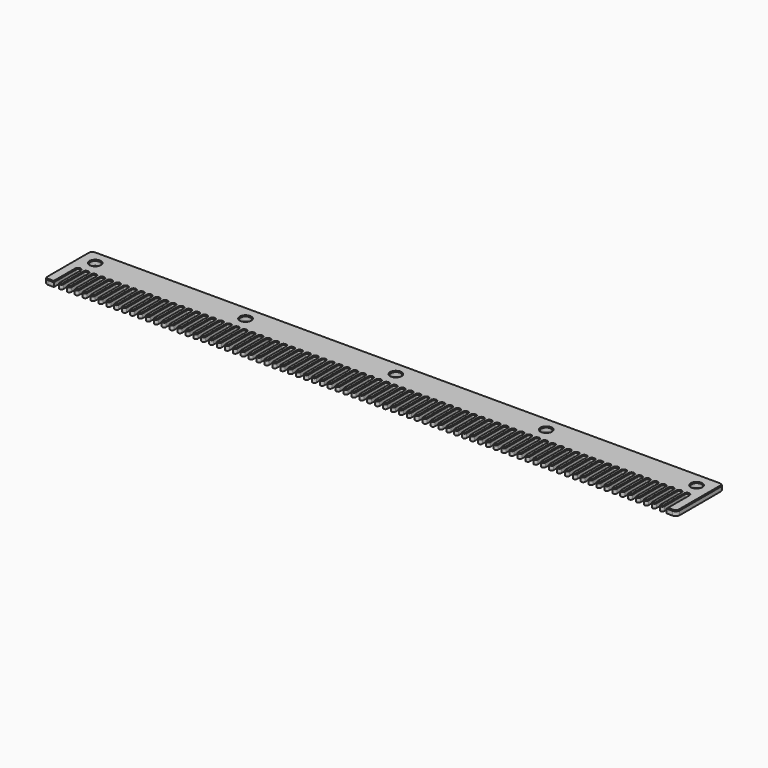
from build123d import *

# Parameters (mm, degrees)
F0_R     = 1.5875
F1_DEPTH = 1.5875
F2_SIZE  = 0.254


# Not quite as in the source:
# - a length typed as a fraction of an inch, garbled in the dataset ("3 / 203.2 mm" for 3/8 in), is restored


with BuildPart() as f1:
    # F0 (on Top) → F1 (new body)
    with BuildSketch(Plane.XY):
        with BuildLine():
            ThreePointArc((101.6, 8.2549999998), (101.2280256121, 9.1530256119), (100.33, 9.5249999998))
            Line((100.33, 9.5249999998), (-100.33, 9.5250000002))
            ThreePointArc((-100.33, 9.5250000002), (-101.2280256121, 9.1530256123), (-101.6, 8.2550000002))
            Line((-101.6, 8.2550000002), (-101.6, -8.255))
            ThreePointArc((-101.6, -8.255), (-101.2280256121, -9.1530256121), (-100.33, -9.525))
            Line((-100.33, -9.525), (-98.425, -9.525))
            Line((-98.425, -9.525), (-98.425, -0.635))
            ThreePointArc((-98.425, -0.635), (-97.79, 0), (-97.155, -0.635))
            Line((-97.155, -0.635), (-97.155, -8.89))
            ThreePointArc((-97.155, -8.89), (-96.52, -9.525), (-95.885, -8.89))
            Line((-95.885, -8.89), (-95.885, -0.635))
            ThreePointArc((-95.885, -0.635), (-95.25, 0), (-94.615, -0.635))
            Line((-94.615, -0.635), (-94.615, -8.89))
            ThreePointArc((-94.615, -8.89), (-93.98, -9.525), (-93.345, -8.89))
            Line((-93.345, -8.89), (-93.345, -0.635))
            ThreePointArc((-93.345, -0.635), (-92.71, 0), (-92.075, -0.635))
            Line((-92.075, -0.635), (-92.075, -8.89))
            ThreePointArc((-92.075, -8.89), (-91.44, -9.525), (-90.805, -8.89))
            Line((-90.805, -8.89), (-90.805, -0.635))
            ThreePointArc((-90.805, -0.635), (-90.17, 0), (-89.535, -0.635))
            Line((-89.535, -0.635), (-89.535, -8.89))
            ThreePointArc((-89.535, -8.89), (-88.9, -9.525), (-88.265, -8.89))
            Line((-88.265, -8.89), (-88.265, -0.635))
            ThreePointArc((-88.265, -0.635), (-87.63, 0), (-86.995, -0.635))
            Line((-86.995, -0.635), (-86.995, -8.89))
            ThreePointArc((-86.995, -8.89), (-86.36, -9.525), (-85.725, -8.89))
            Line((-85.725, -8.89), (-85.725, -0.635))
            ThreePointArc((-85.725, -0.635), (-85.09, 0), (-84.455, -0.635))
            Line((-84.455, -0.635), (-84.455, -8.89))
            ThreePointArc((-84.455, -8.89), (-83.82, -9.525), (-83.185, -8.89))
            Line((-83.185, -8.89), (-83.185, -0.635))
            ThreePointArc((-83.185, -0.635), (-82.55, 0), (-81.915, -0.635))
            Line((-81.915, -0.635), (-81.915, -8.89))
            ThreePointArc((-81.915, -8.89), (-81.28, -9.525), (-80.645, -8.89))
            Line((-80.645, -8.89), (-80.645, -0.635))
            ThreePointArc((-80.645, -0.635), (-80.01, 0), (-79.375, -0.635))
            Line((-79.375, -0.635), (-79.375, -8.89))
            ThreePointArc((-79.375, -8.89), (-78.74, -9.525), (-78.105, -8.89))
            Line((-78.105, -8.89), (-78.105, -0.635))
            ThreePointArc((-78.105, -0.635), (-77.47, 0), (-76.835, -0.635))
            Line((-76.835, -0.635), (-76.835, -8.89))
            ThreePointArc((-76.835, -8.89), (-76.2, -9.525), (-75.565, -8.89))
            Line((-75.565, -8.89), (-75.565, -0.635))
            ThreePointArc((-75.565, -0.635), (-74.93, 0), (-74.295, -0.635))
            Line((-74.295, -0.635), (-74.295, -8.89))
            ThreePointArc((-74.295, -8.89), (-73.66, -9.525), (-73.025, -8.89))
            Line((-73.025, -8.89), (-73.025, -0.635))
            ThreePointArc((-73.025, -0.635), (-72.39, 0), (-71.755, -0.635))
            Line((-71.755, -0.635), (-71.755, -8.89))
            ThreePointArc((-71.755, -8.89), (-71.12, -9.525), (-70.485, -8.89))
            Line((-70.485, -8.89), (-70.485, -0.635))
            ThreePointArc((-70.485, -0.635), (-69.85, 0), (-69.215, -0.635))
            Line((-69.215, -0.635), (-69.215, -8.89))
            ThreePointArc((-69.215, -8.89), (-68.58, -9.525), (-67.945, -8.89))
            Line((-67.945, -8.89), (-67.945, -0.635))
            ThreePointArc((-67.945, -0.635), (-67.31, 0), (-66.675, -0.635))
            Line((-66.675, -0.635), (-66.675, -8.89))
            ThreePointArc((-66.675, -8.89), (-66.04, -9.525), (-65.405, -8.89))
            Line((-65.405, -8.89), (-65.405, -0.635))
            ThreePointArc((-65.405, -0.635), (-64.77, 0), (-64.135, -0.635))
            Line((-64.135, -0.635), (-64.135, -8.89))
            ThreePointArc((-64.135, -8.89), (-63.5, -9.525), (-62.865, -8.89))
            Line((-62.865, -8.89), (-62.865, -0.635))
            ThreePointArc((-62.865, -0.635), (-62.23, 0), (-61.595, -0.635))
            Line((-61.595, -0.635), (-61.595, -8.89))
            ThreePointArc((-61.595, -8.89), (-60.96, -9.525), (-60.325, -8.89))
            Line((-60.325, -8.89), (-60.325, -0.635))
            ThreePointArc((-60.325, -0.635), (-59.69, 0), (-59.055, -0.635))
            Line((-59.055, -0.635), (-59.055, -8.89))
            ThreePointArc((-59.055, -8.89), (-58.42, -9.525), (-57.785, -8.89))
            Line((-57.785, -8.89), (-57.785, -0.635))
            ThreePointArc((-57.785, -0.635), (-57.15, 0), (-56.515, -0.635))
            Line((-56.515, -0.635), (-56.515, -8.89))
            ThreePointArc((-56.515, -8.89), (-55.88, -9.525), (-55.245, -8.89))
            Line((-55.245, -8.89), (-55.245, -0.635))
            ThreePointArc((-55.245, -0.635), (-54.61, 0), (-53.975, -0.635))
            Line((-53.975, -0.635), (-53.975, -8.89))
            ThreePointArc((-53.975, -8.89), (-53.34, -9.525), (-52.705, -8.89))
            Line((-52.705, -8.89), (-52.705, -0.635))
            ThreePointArc((-52.705, -0.635), (-52.07, 0), (-51.435, -0.635))
            Line((-51.435, -0.635), (-51.435, -8.89))
            ThreePointArc((-51.435, -8.89), (-50.8, -9.525), (-50.165, -8.89))
            Line((-50.165, -8.89), (-50.165, -0.635))
            ThreePointArc((-50.165, -0.635), (-49.53, 0), (-48.895, -0.635))
            Line((-48.895, -0.635), (-48.895, -8.89))
            ThreePointArc((-48.895, -8.89), (-48.26, -9.525), (-47.625, -8.89))
            Line((-47.625, -8.89), (-47.625, -0.635))
            ThreePointArc((-47.625, -0.635), (-46.99, 0), (-46.355, -0.635))
            Line((-46.355, -0.635), (-46.355, -8.89))
            ThreePointArc((-46.355, -8.89), (-45.72, -9.525), (-45.085, -8.89))
            Line((-45.085, -8.89), (-45.085, -0.635))
            ThreePointArc((-45.085, -0.635), (-44.45, 0), (-43.815, -0.635))
            Line((-43.815, -0.635), (-43.815, -8.89))
            ThreePointArc((-43.815, -8.89), (-43.18, -9.525), (-42.545, -8.89))
            Line((-42.545, -8.89), (-42.545, -0.635))
            ThreePointArc((-42.545, -0.635), (-41.91, 0), (-41.275, -0.635))
            Line((-41.275, -0.635), (-41.275, -8.89))
            ThreePointArc((-41.275, -8.89), (-40.64, -9.525), (-40.005, -8.89))
            Line((-40.005, -8.89), (-40.005, -0.635))
            ThreePointArc((-40.005, -0.635), (-39.37, 0), (-38.735, -0.635))
            Line((-38.735, -0.635), (-38.735, -8.89))
            ThreePointArc((-38.735, -8.89), (-38.1, -9.525), (-37.465, -8.89))
            Line((-37.465, -8.89), (-37.465, -0.635))
            ThreePointArc((-37.465, -0.635), (-36.83, 0), (-36.195, -0.635))
            Line((-36.195, -0.635), (-36.195, -8.89))
            ThreePointArc((-36.195, -8.89), (-35.56, -9.525), (-34.925, -8.89))
            Line((-34.925, -8.89), (-34.925, -0.635))
            ThreePointArc((-34.925, -0.635), (-34.29, 0), (-33.655, -0.635))
            Line((-33.655, -0.635), (-33.655, -8.89))
            ThreePointArc((-33.655, -8.89), (-33.02, -9.525), (-32.385, -8.89))
            Line((-32.385, -8.89), (-32.385, -0.635))
            ThreePointArc((-32.385, -0.635), (-31.75, 0), (-31.115, -0.635))
            Line((-31.115, -0.635), (-31.115, -8.89))
            ThreePointArc((-31.115, -8.89), (-30.48, -9.525), (-29.845, -8.89))
            Line((-29.845, -8.89), (-29.845, -0.635))
            ThreePointArc((-29.845, -0.635), (-29.21, 0), (-28.575, -0.635))
            Line((-28.575, -0.635), (-28.575, -8.89))
            ThreePointArc((-28.575, -8.89), (-27.94, -9.525), (-27.305, -8.89))
            Line((-27.305, -8.89), (-27.305, -0.635))
            ThreePointArc((-27.305, -0.635), (-26.67, 0), (-26.035, -0.635))
            Line((-26.035, -0.635), (-26.035, -8.89))
            ThreePointArc((-26.035, -8.89), (-25.4, -9.525), (-24.765, -8.89))
            Line((-24.765, -8.89), (-24.765, -0.635))
            ThreePointArc((-24.765, -0.635), (-24.13, 0), (-23.495, -0.635))
            Line((-23.495, -0.635), (-23.495, -8.89))
            ThreePointArc((-23.495, -8.89), (-22.86, -9.525), (-22.225, -8.89))
            Line((-22.225, -8.89), (-22.225, -0.635))
            ThreePointArc((-22.225, -0.635), (-21.59, 0), (-20.955, -0.635))
            Line((-20.955, -0.635), (-20.955, -8.89))
            ThreePointArc((-20.955, -8.89), (-20.32, -9.525), (-19.685, -8.89))
            Line((-19.685, -8.89), (-19.685, -0.635))
            ThreePointArc((-19.685, -0.635), (-19.05, 0), (-18.415, -0.635))
            Line((-18.415, -0.635), (-18.415, -8.89))
            ThreePointArc((-18.415, -8.89), (-17.78, -9.525), (-17.145, -8.89))
            Line((-17.145, -8.89), (-17.145, -0.635))
            ThreePointArc((-17.145, -0.635), (-16.51, 0), (-15.875, -0.635))
            Line((-15.875, -0.635), (-15.875, -8.89))
            ThreePointArc((-15.875, -8.89), (-15.24, -9.525), (-14.605, -8.89))
            Line((-14.605, -8.89), (-14.605, -0.635))
            ThreePointArc((-14.605, -0.635), (-13.97, 0), (-13.335, -0.635))
            Line((-13.335, -0.635), (-13.335, -8.89))
            ThreePointArc((-13.335, -8.89), (-12.7, -9.525), (-12.065, -8.89))
            Line((-12.065, -8.89), (-12.065, -0.635))
            ThreePointArc((-12.065, -0.635), (-11.43, 0), (-10.795, -0.635))
            Line((-10.795, -0.635), (-10.795, -8.89))
            ThreePointArc((-10.795, -8.89), (-10.16, -9.525), (-9.525, -8.89))
            Line((-9.525, -8.89), (-9.525, -0.635))
            ThreePointArc((-9.525, -0.635), (-8.89, 0), (-8.255, -0.635))
            Line((-8.255, -0.635), (-8.255, -8.89))
            ThreePointArc((-8.255, -8.89), (-7.62, -9.525), (-6.985, -8.89))
            Line((-6.985, -8.89), (-6.985, -0.635))
            ThreePointArc((-6.985, -0.635), (-6.35, 0), (-5.715, -0.635))
            Line((-5.715, -0.635), (-5.715, -8.89))
            ThreePointArc((-5.715, -8.89), (-5.08, -9.525), (-4.445, -8.89))
            Line((-4.445, -8.89), (-4.445, -0.635))
            ThreePointArc((-4.445, -0.635), (-3.81, 0), (-3.175, -0.635))
            Line((-3.175, -0.635), (-3.175, -8.89))
            ThreePointArc((-3.175, -8.89), (-2.54, -9.525), (-1.905, -8.89))
            Line((-1.905, -8.89), (-1.905, -0.635))
            ThreePointArc((-1.905, -0.635), (-1.27, 0), (-0.635, -0.635))
            Line((-0.635, -0.635), (-0.635, -8.89))
            ThreePointArc((-0.635, -8.89), (0, -9.525), (0.635, -8.89))
            Line((0.635, -8.89), (0.635, -0.635))
            ThreePointArc((0.635, -0.635), (1.27, 0), (1.905, -0.635))
            Line((1.905, -0.635), (1.905, -8.89))
            ThreePointArc((1.905, -8.89), (2.54, -9.525), (3.175, -8.89))
            Line((3.175, -8.89), (3.175, -0.635))
            ThreePointArc((3.175, -0.635), (3.81, 0), (4.445, -0.635))
            Line((4.445, -0.635), (4.445, -8.89))
            ThreePointArc((4.445, -8.89), (5.08, -9.525), (5.715, -8.89))
            Line((5.715, -8.89), (5.715, -0.635))
            ThreePointArc((5.715, -0.635), (6.35, 0), (6.985, -0.635))
            Line((6.985, -0.635), (6.985, -8.89))
            ThreePointArc((6.985, -8.89), (7.62, -9.525), (8.255, -8.89))
            Line((8.255, -8.89), (8.255, -0.635))
            ThreePointArc((8.255, -0.635), (8.89, 0), (9.525, -0.635))
            Line((9.525, -0.635), (9.525, -8.89))
            ThreePointArc((9.525, -8.89), (10.16, -9.525), (10.795, -8.89))
            Line((10.795, -8.89), (10.795, -0.635))
            ThreePointArc((10.795, -0.635), (11.43, 0), (12.065, -0.635))
            Line((12.065, -0.635), (12.065, -8.89))
            ThreePointArc((12.065, -8.89), (12.7, -9.525), (13.335, -8.89))
            Line((13.335, -8.89), (13.335, -0.635))
            ThreePointArc((13.335, -0.635), (13.97, 0), (14.605, -0.635))
            Line((14.605, -0.635), (14.605, -8.89))
            ThreePointArc((14.605, -8.89), (15.24, -9.525), (15.875, -8.89))
            Line((15.875, -8.89), (15.875, -0.635))
            ThreePointArc((15.875, -0.635), (16.51, 0), (17.145, -0.635))
            Line((17.145, -0.635), (17.145, -8.89))
            ThreePointArc((17.145, -8.89), (17.78, -9.525), (18.415, -8.89))
            Line((18.415, -8.89), (18.415, -0.635))
            ThreePointArc((18.415, -0.635), (19.05, 0), (19.685, -0.635))
            Line((19.685, -0.635), (19.685, -8.89))
            ThreePointArc((19.685, -8.89), (20.32, -9.525), (20.955, -8.89))
            Line((20.955, -8.89), (20.955, -0.635))
            ThreePointArc((20.955, -0.635), (21.59, 0), (22.225, -0.635))
            Line((22.225, -0.635), (22.225, -8.89))
            ThreePointArc((22.225, -8.89), (22.86, -9.525), (23.495, -8.89))
            Line((23.495, -8.89), (23.495, -0.635))
            ThreePointArc((23.495, -0.635), (24.13, 0), (24.765, -0.635))
            Line((24.765, -0.635), (24.765, -8.89))
            ThreePointArc((24.765, -8.89), (25.4, -9.525), (26.035, -8.89))
            Line((26.035, -8.89), (26.035, -0.635))
            ThreePointArc((26.035, -0.635), (26.67, 0), (27.305, -0.635))
            Line((27.305, -0.635), (27.305, -8.89))
            ThreePointArc((27.305, -8.89), (27.94, -9.525), (28.575, -8.89))
            Line((28.575, -8.89), (28.575, -0.635))
            ThreePointArc((28.575, -0.635), (29.21, 0), (29.845, -0.635))
            Line((29.845, -0.635), (29.845, -8.89))
            ThreePointArc((29.845, -8.89), (30.48, -9.525), (31.115, -8.89))
            Line((31.115, -8.89), (31.115, -0.635))
            ThreePointArc((31.115, -0.635), (31.75, 0), (32.385, -0.635))
            Line((32.385, -0.635), (32.385, -8.89))
            ThreePointArc((32.385, -8.89), (33.02, -9.525), (33.655, -8.89))
            Line((33.655, -8.89), (33.655, -0.635))
            ThreePointArc((33.655, -0.635), (34.29, 0), (34.925, -0.635))
            Line((34.925, -0.635), (34.925, -8.89))
            ThreePointArc((34.925, -8.89), (35.56, -9.525), (36.195, -8.89))
            Line((36.195, -8.89), (36.195, -0.635))
            ThreePointArc((36.195, -0.635), (36.83, 0), (37.465, -0.635))
            Line((37.465, -0.635), (37.465, -8.89))
            ThreePointArc((37.465, -8.89), (38.1, -9.525), (38.735, -8.89))
            Line((38.735, -8.89), (38.735, -0.635))
            ThreePointArc((38.735, -0.635), (39.37, 0), (40.005, -0.635))
            Line((40.005, -0.635), (40.005, -8.89))
            ThreePointArc((40.005, -8.89), (40.64, -9.525), (41.275, -8.89))
            Line((41.275, -8.89), (41.275, -0.635))
            ThreePointArc((41.275, -0.635), (41.91, 0), (42.545, -0.635))
            Line((42.545, -0.635), (42.545, -8.89))
            ThreePointArc((42.545, -8.89), (43.18, -9.525), (43.815, -8.89))
            Line((43.815, -8.89), (43.815, -0.635))
            ThreePointArc((43.815, -0.635), (44.45, 0), (45.085, -0.635))
            Line((45.085, -0.635), (45.085, -8.89))
            ThreePointArc((45.085, -8.89), (45.72, -9.525), (46.355, -8.89))
            Line((46.355, -8.89), (46.355, -0.635))
            ThreePointArc((46.355, -0.635), (46.99, 0), (47.625, -0.635))
            Line((47.625, -0.635), (47.625, -8.89))
            ThreePointArc((47.625, -8.89), (48.26, -9.525), (48.895, -8.89))
            Line((48.895, -8.89), (48.895, -0.635))
            ThreePointArc((48.895, -0.635), (49.53, 0), (50.165, -0.635))
            Line((50.165, -0.635), (50.165, -8.89))
            ThreePointArc((50.165, -8.89), (50.8, -9.525), (51.435, -8.89))
            Line((51.435, -8.89), (51.435, -0.635))
            ThreePointArc((51.435, -0.635), (52.07, 0), (52.705, -0.635))
            Line((52.705, -0.635), (52.705, -8.89))
            ThreePointArc((52.705, -8.89), (53.34, -9.525), (53.975, -8.89))
            Line((53.975, -8.89), (53.975, -0.635))
            ThreePointArc((53.975, -0.635), (54.61, 0), (55.245, -0.635))
            Line((55.245, -0.635), (55.245, -8.89))
            ThreePointArc((55.245, -8.89), (55.88, -9.525), (56.515, -8.89))
            Line((56.515, -8.89), (56.515, -0.635))
            ThreePointArc((56.515, -0.635), (57.15, 0), (57.785, -0.635))
            Line((57.785, -0.635), (57.785, -8.89))
            ThreePointArc((57.785, -8.89), (58.42, -9.525), (59.055, -8.89))
            Line((59.055, -8.89), (59.055, -0.635))
            ThreePointArc((59.055, -0.635), (59.69, 0), (60.325, -0.635))
            Line((60.325, -0.635), (60.325, -8.89))
            ThreePointArc((60.325, -8.89), (60.96, -9.525), (61.595, -8.89))
            Line((61.595, -8.89), (61.595, -0.635))
            ThreePointArc((61.595, -0.635), (62.23, 0), (62.865, -0.635))
            Line((62.865, -0.635), (62.865, -8.89))
            ThreePointArc((62.865, -8.89), (63.5, -9.525), (64.135, -8.89))
            Line((64.135, -8.89), (64.135, -0.635))
            ThreePointArc((64.135, -0.635), (64.77, 0), (65.405, -0.635))
            Line((65.405, -0.635), (65.405, -8.89))
            ThreePointArc((65.405, -8.89), (66.04, -9.525), (66.675, -8.89))
            Line((66.675, -8.89), (66.675, -0.635))
            ThreePointArc((66.675, -0.635), (67.31, 0), (67.945, -0.635))
            Line((67.945, -0.635), (67.945, -8.89))
            ThreePointArc((67.945, -8.89), (68.58, -9.525), (69.215, -8.89))
            Line((69.215, -8.89), (69.215, -0.635))
            ThreePointArc((69.215, -0.635), (69.85, 0), (70.485, -0.635))
            Line((70.485, -0.635), (70.485, -8.89))
            ThreePointArc((70.485, -8.89), (71.12, -9.525), (71.755, -8.89))
            Line((71.755, -8.89), (71.755, -0.635))
            ThreePointArc((71.755, -0.635), (72.39, 0), (73.025, -0.635))
            Line((73.025, -0.635), (73.025, -8.89))
            ThreePointArc((73.025, -8.89), (73.66, -9.525), (74.295, -8.89))
            Line((74.295, -8.89), (74.295, -0.635))
            ThreePointArc((74.295, -0.635), (74.93, 0), (75.565, -0.635))
            Line((75.565, -0.635), (75.565, -8.89))
            ThreePointArc((75.565, -8.89), (76.2, -9.525), (76.835, -8.89))
            Line((76.835, -8.89), (76.835, -0.635))
            ThreePointArc((76.835, -0.635), (77.47, 0), (78.105, -0.635))
            Line((78.105, -0.635), (78.105, -8.89))
            ThreePointArc((78.105, -8.89), (78.74, -9.525), (79.375, -8.89))
            Line((79.375, -8.89), (79.375, -0.635))
            ThreePointArc((79.375, -0.635), (80.01, 0), (80.645, -0.635))
            Line((80.645, -0.635), (80.645, -8.89))
            ThreePointArc((80.645, -8.89), (81.28, -9.525), (81.915, -8.89))
            Line((81.915, -8.89), (81.915, -0.635))
            ThreePointArc((81.915, -0.635), (82.55, 0), (83.185, -0.635))
            Line((83.185, -0.635), (83.185, -8.89))
            ThreePointArc((83.185, -8.89), (83.82, -9.525), (84.455, -8.89))
            Line((84.455, -8.89), (84.455, -0.635))
            ThreePointArc((84.455, -0.635), (85.09, 0), (85.725, -0.635))
            Line((85.725, -0.635), (85.725, -8.89))
            ThreePointArc((85.725, -8.89), (86.36, -9.525), (86.995, -8.89))
            Line((86.995, -8.89), (86.995, -0.635))
            ThreePointArc((86.995, -0.635), (87.63, 0), (88.265, -0.635))
            Line((88.265, -0.635), (88.265, -8.89))
            ThreePointArc((88.265, -8.89), (88.9, -9.525), (89.535, -8.89))
            Line((89.535, -8.89), (89.535, -0.635))
            ThreePointArc((89.535, -0.635), (90.17, 0), (90.805, -0.635))
            Line((90.805, -0.635), (90.805, -8.89))
            ThreePointArc((90.805, -8.89), (91.44, -9.525), (92.075, -8.89))
            Line((92.075, -8.89), (92.075, -0.635))
            ThreePointArc((92.075, -0.635), (92.71, 0), (93.345, -0.635))
            Line((93.345, -0.635), (93.345, -8.89))
            ThreePointArc((93.345, -8.89), (93.98, -9.525), (94.615, -8.89))
            Line((94.615, -8.89), (94.615, -0.635))
            ThreePointArc((94.615, -0.635), (95.25, 0), (95.885, -0.635))
            Line((95.885, -0.635), (95.885, -8.89))
            ThreePointArc((95.885, -8.89), (96.52, -9.525), (97.155, -8.89))
            Line((97.155, -8.89), (97.155, -0.635))
            ThreePointArc((97.155, -0.635), (97.7896726274, -0.0003273725), (98.4243452549, -0.635))
            Line((98.4243452549, -0.635), (98.4243452549, -9.525))
            Line((98.4243452549, -9.525), (100.33, -9.525))
            ThreePointArc((100.33, -9.525), (101.2280256121, -9.1530256121), (101.6, -8.255))
            Line((101.6, -8.255), (101.6, 8.2549999998))
        make_face()
        with Locations((-96.6, 4.7625)):
            Circle(F0_R, mode=Mode.SUBTRACT)
        with Locations((-48.3, 4.7625)):
            Circle(F0_R, mode=Mode.SUBTRACT)
        with Locations((0, 4.7625)):
            Circle(F0_R, mode=Mode.SUBTRACT)
        with Locations((48.3, 4.7625)):
            Circle(F0_R, mode=Mode.SUBTRACT)
        with Locations((96.6, 4.7625)):
            Circle(F0_R, mode=Mode.SUBTRACT)
    extrude(amount=F1_DEPTH)

    # F2
    f2_edges = [f1.edges().sort_by_distance(p)[0] for p in [
        (101.228026, -9.153026, 1.5875),
        (101.6, 0, 1.5875),
        (101.228026, 9.153026, 1.5875),
        (0, 9.525, 1.5875),
        (-101.228026, 9.153026, 1.5875),
        (-101.6, 0, 1.5875),
        (-101.228026, -9.153026, 1.5875),
        (-99.3775, -9.525, 1.5875),
        (-98.425, -5.08, 1.5875),
        (-97.79, 0, 1.5875),
        (-97.155, -4.7625, 1.5875),
        (-96.52, -9.525, 1.5875),
        (-95.885, -4.7625, 1.5875),
        (-95.25, 0, 1.5875),
        (-94.615, -4.7625, 1.5875),
        (-93.98, -9.525, 1.5875),
        (-93.345, -4.7625, 1.5875),
        (-92.71, 0, 1.5875),
        (-92.075, -4.7625, 1.5875),
        (-91.44, -9.525, 1.5875),
        (-90.805, -4.7625, 1.5875),
        (-90.17, 0, 1.5875),
        (-89.535, -4.7625, 1.5875),
        (-88.9, -9.525, 1.5875),
        (-88.265, -4.7625, 1.5875),
        (-87.63, 0, 1.5875),
        (-86.995, -4.7625, 1.5875),
        (-86.36, -9.525, 1.5875),
        (-85.725, -4.7625, 1.5875),
        (-85.09, 0, 1.5875),
        (-84.455, -4.7625, 1.5875),
        (-83.82, -9.525, 1.5875),
        (-83.185, -4.7625, 1.5875),
        (-82.55, 0, 1.5875),
        (-81.915, -4.7625, 1.5875),
        (-81.28, -9.525, 1.5875),
        (-80.645, -4.7625, 1.5875),
        (-80.01, 0, 1.5875),
        (-79.375, -4.7625, 1.5875),
        (-78.74, -9.525, 1.5875),
        (-78.105, -4.7625, 1.5875),
        (-77.47, 0, 1.5875),
        (-76.835, -4.7625, 1.5875),
        (-76.2, -9.525, 1.5875),
        (-75.565, -4.7625, 1.5875),
        (-74.93, 0, 1.5875),
        (-74.295, -4.7625, 1.5875),
        (-73.66, -9.525, 1.5875),
        (-73.025, -4.7625, 1.5875),
        (-72.39, 0, 1.5875),
        (-71.755, -4.7625, 1.5875),
        (-71.12, -9.525, 1.5875),
        (-70.485, -4.7625, 1.5875),
        (-69.85, 0, 1.5875),
        (-69.215, -4.7625, 1.5875),
        (-68.58, -9.525, 1.5875),
        (-67.945, -4.7625, 1.5875),
        (-67.31, 0, 1.5875),
        (-66.675, -4.7625, 1.5875),
        (-66.04, -9.525, 1.5875),
        (-65.405, -4.7625, 1.5875),
        (-64.77, 0, 1.5875),
        (-64.135, -4.7625, 1.5875),
        (-63.5, -9.525, 1.5875),
        (-62.865, -4.7625, 1.5875),
        (-62.23, 0, 1.5875),
        (-61.595, -4.7625, 1.5875),
        (-60.96, -9.525, 1.5875),
        (-60.325, -4.7625, 1.5875),
        (-59.69, 0, 1.5875),
        (-59.055, -4.7625, 1.5875),
        (-58.42, -9.525, 1.5875),
        (-57.785, -4.7625, 1.5875),
        (-57.15, 0, 1.5875),
        (-56.515, -4.7625, 1.5875),
        (-55.88, -9.525, 1.5875),
        (-55.245, -4.7625, 1.5875),
        (-54.61, 0, 1.5875),
        (-53.975, -4.7625, 1.5875),
        (-53.34, -9.525, 1.5875),
        (-52.705, -4.7625, 1.5875),
        (-52.07, 0, 1.5875),
        (-51.435, -4.7625, 1.5875),
        (-50.8, -9.525, 1.5875),
        (-50.165, -4.7625, 1.5875),
        (-49.53, 0, 1.5875),
        (-48.895, -4.7625, 1.5875),
        (-48.26, -9.525, 1.5875),
        (-47.625, -4.7625, 1.5875),
        (-46.99, 0, 1.5875),
        (-46.355, -4.7625, 1.5875),
        (-45.72, -9.525, 1.5875),
        (-45.085, -4.7625, 1.5875),
        (-44.45, 0, 1.5875),
        (-43.815, -4.7625, 1.5875),
        (-43.18, -9.525, 1.5875),
        (-42.545, -4.7625, 1.5875),
        (-41.91, 0, 1.5875),
        (-41.275, -4.7625, 1.5875),
        (-40.64, -9.525, 1.5875),
        (-40.005, -4.7625, 1.5875),
        (-39.37, 0, 1.5875),
        (-38.735, -4.7625, 1.5875),
        (-38.1, -9.525, 1.5875),
        (-37.465, -4.7625, 1.5875),
        (-36.83, 0, 1.5875),
        (-36.195, -4.7625, 1.5875),
        (-35.56, -9.525, 1.5875),
        (-34.925, -4.7625, 1.5875),
        (-34.29, 0, 1.5875),
        (-33.655, -4.7625, 1.5875),
        (-33.02, -9.525, 1.5875),
        (-32.385, -4.7625, 1.5875),
        (-31.75, 0, 1.5875),
        (-31.115, -4.7625, 1.5875),
        (-30.48, -9.525, 1.5875),
        (-29.845, -4.7625, 1.5875),
        (-29.21, 0, 1.5875),
        (-28.575, -4.7625, 1.5875),
        (-27.94, -9.525, 1.5875),
        (-27.305, -4.7625, 1.5875),
        (-26.67, 0, 1.5875),
        (-26.035, -4.7625, 1.5875),
        (-25.4, -9.525, 1.5875),
        (-24.765, -4.7625, 1.5875),
        (-24.13, 0, 1.5875),
        (-23.495, -4.7625, 1.5875),
        (-22.86, -9.525, 1.5875),
        (-22.225, -4.7625, 1.5875),
        (-21.59, 0, 1.5875),
        (-20.955, -4.7625, 1.5875),
        (-20.32, -9.525, 1.5875),
        (-19.685, -4.7625, 1.5875),
        (-19.05, 0, 1.5875),
        (-18.415, -4.7625, 1.5875),
        (-17.78, -9.525, 1.5875),
        (-17.145, -4.7625, 1.5875),
        (-16.51, 0, 1.5875),
        (-15.875, -4.7625, 1.5875),
        (-15.24, -9.525, 1.5875),
        (-14.605, -4.7625, 1.5875),
        (-13.97, 0, 1.5875),
        (-13.335, -4.7625, 1.5875),
        (-12.7, -9.525, 1.5875),
        (-12.065, -4.7625, 1.5875),
        (-11.43, 0, 1.5875),
        (-10.795, -4.7625, 1.5875),
        (-10.16, -9.525, 1.5875),
        (-9.525, -4.7625, 1.5875),
        (-8.89, 0, 1.5875),
        (-8.255, -4.7625, 1.5875),
        (-7.62, -9.525, 1.5875),
        (-6.985, -4.7625, 1.5875),
        (-6.35, 0, 1.5875),
        (-5.715, -4.7625, 1.5875),
        (-5.08, -9.525, 1.5875),
        (-4.445, -4.7625, 1.5875),
        (-3.81, 0, 1.5875),
        (-3.175, -4.7625, 1.5875),
        (-2.54, -9.525, 1.5875),
        (-1.905, -4.7625, 1.5875),
        (-1.27, 0, 1.5875),
        (-0.635, -4.7625, 1.5875),
        (0, -9.525, 1.5875),
        (0.635, -4.7625, 1.5875),
        (1.27, 0, 1.5875),
        (1.905, -4.7625, 1.5875),
        (2.54, -9.525, 1.5875),
        (3.175, -4.7625, 1.5875),
        (3.81, 0, 1.5875),
        (4.445, -4.7625, 1.5875),
        (5.08, -9.525, 1.5875),
        (5.715, -4.7625, 1.5875),
        (6.35, 0, 1.5875),
        (6.985, -4.7625, 1.5875),
        (7.62, -9.525, 1.5875),
        (8.255, -4.7625, 1.5875),
        (8.89, 0, 1.5875),
        (9.525, -4.7625, 1.5875),
        (10.16, -9.525, 1.5875),
        (10.795, -4.7625, 1.5875),
        (11.43, 0, 1.5875),
        (12.065, -4.7625, 1.5875),
        (12.7, -9.525, 1.5875),
        (13.335, -4.7625, 1.5875),
        (13.97, 0, 1.5875),
        (14.605, -4.7625, 1.5875),
        (15.24, -9.525, 1.5875),
        (15.875, -4.7625, 1.5875),
        (16.51, 0, 1.5875),
        (17.145, -4.7625, 1.5875),
        (17.78, -9.525, 1.5875),
        (18.415, -4.7625, 1.5875),
        (19.05, 0, 1.5875),
        (19.685, -4.7625, 1.5875),
        (20.32, -9.525, 1.5875),
        (20.955, -4.7625, 1.5875),
        (21.59, 0, 1.5875),
        (22.225, -4.7625, 1.5875),
        (22.86, -9.525, 1.5875),
        (23.495, -4.7625, 1.5875),
        (24.13, 0, 1.5875),
        (24.765, -4.7625, 1.5875),
        (25.4, -9.525, 1.5875),
        (26.035, -4.7625, 1.5875),
        (26.67, 0, 1.5875),
        (27.305, -4.7625, 1.5875),
        (27.94, -9.525, 1.5875),
        (28.575, -4.7625, 1.5875),
        (29.21, 0, 1.5875),
        (29.845, -4.7625, 1.5875),
        (30.48, -9.525, 1.5875),
        (31.115, -4.7625, 1.5875),
        (31.75, 0, 1.5875),
        (32.385, -4.7625, 1.5875),
        (33.02, -9.525, 1.5875),
        (33.655, -4.7625, 1.5875),
        (34.29, 0, 1.5875),
        (34.925, -4.7625, 1.5875),
        (35.56, -9.525, 1.5875),
        (36.195, -4.7625, 1.5875),
        (36.83, 0, 1.5875),
        (37.465, -4.7625, 1.5875),
        (38.1, -9.525, 1.5875),
        (38.735, -4.7625, 1.5875),
        (39.37, 0, 1.5875),
        (40.005, -4.7625, 1.5875),
        (40.64, -9.525, 1.5875),
        (41.275, -4.7625, 1.5875),
        (41.91, 0, 1.5875),
        (42.545, -4.7625, 1.5875),
        (43.18, -9.525, 1.5875),
        (43.815, -4.7625, 1.5875),
        (44.45, 0, 1.5875),
        (45.085, -4.7625, 1.5875),
        (45.72, -9.525, 1.5875),
        (46.355, -4.7625, 1.5875),
        (46.99, 0, 1.5875),
        (47.625, -4.7625, 1.5875),
        (48.26, -9.525, 1.5875),
        (48.895, -4.7625, 1.5875),
        (49.53, 0, 1.5875),
        (50.165, -4.7625, 1.5875),
        (50.8, -9.525, 1.5875),
        (51.435, -4.7625, 1.5875),
        (52.07, 0, 1.5875),
        (52.705, -4.7625, 1.5875),
        (53.34, -9.525, 1.5875),
        (53.975, -4.7625, 1.5875),
        (54.61, 0, 1.5875),
        (55.245, -4.7625, 1.5875),
        (55.88, -9.525, 1.5875),
        (56.515, -4.7625, 1.5875),
        (57.15, 0, 1.5875),
        (57.785, -4.7625, 1.5875),
        (58.42, -9.525, 1.5875),
        (59.055, -4.7625, 1.5875),
        (59.69, 0, 1.5875),
        (60.325, -4.7625, 1.5875),
        (60.96, -9.525, 1.5875),
        (61.595, -4.7625, 1.5875),
        (62.23, 0, 1.5875),
        (62.865, -4.7625, 1.5875),
        (63.5, -9.525, 1.5875),
        (64.135, -4.7625, 1.5875),
        (64.77, 0, 1.5875),
        (65.405, -4.7625, 1.5875),
        (66.04, -9.525, 1.5875),
        (66.675, -4.7625, 1.5875),
        (67.31, 0, 1.5875),
        (67.945, -4.7625, 1.5875),
        (68.58, -9.525, 1.5875),
        (69.215, -4.7625, 1.5875),
        (69.85, 0, 1.5875),
        (70.485, -4.7625, 1.5875),
        (71.12, -9.525, 1.5875),
        (71.755, -4.7625, 1.5875),
        (72.39, 0, 1.5875),
        (73.025, -4.7625, 1.5875),
        (73.66, -9.525, 1.5875),
        (74.295, -4.7625, 1.5875),
        (74.93, 0, 1.5875),
        (75.565, -4.7625, 1.5875),
        (76.2, -9.525, 1.5875),
        (76.835, -4.7625, 1.5875),
        (77.47, 0, 1.5875),
        (78.105, -4.7625, 1.5875),
        (78.74, -9.525, 1.5875),
        (79.375, -4.7625, 1.5875),
        (80.01, 0, 1.5875),
        (80.645, -4.7625, 1.5875),
        (81.28, -9.525, 1.5875),
        (81.915, -4.7625, 1.5875),
        (82.55, 0, 1.5875),
        (83.185, -4.7625, 1.5875),
        (83.82, -9.525, 1.5875),
        (84.455, -4.7625, 1.5875),
        (85.09, 0, 1.5875),
        (85.725, -4.7625, 1.5875),
        (86.36, -9.525, 1.5875),
        (86.995, -4.7625, 1.5875),
        (87.63, 0, 1.5875),
        (88.265, -4.7625, 1.5875),
        (88.9, -9.525, 1.5875),
        (89.535, -4.7625, 1.5875),
        (90.17, 0, 1.5875),
        (90.805, -4.7625, 1.5875),
        (91.44, -9.525, 1.5875),
        (92.075, -4.7625, 1.5875),
        (92.71, 0, 1.5875),
        (93.345, -4.7625, 1.5875),
        (93.98, -9.525, 1.5875),
        (94.615, -4.7625, 1.5875),
        (95.25, 0, 1.5875),
        (95.885, -4.7625, 1.5875),
        (96.52, -9.525, 1.5875),
        (97.155, -4.7625, 1.5875),
        (97.789673, -0.000327, 1.5875),
        (98.424345, -5.08, 1.5875),
        (99.377173, -9.525, 1.5875),
        (-98.1875, 4.7625, 1.5875),
        (-49.8875, 4.7625, 1.5875),
        (-1.5875, 4.7625, 1.5875),
        (46.7125, 4.7625, 1.5875),
        (95.0125, 4.7625, 1.5875),
    ]]
    chamfer(f2_edges, length=F2_SIZE)


solid = f1.part
